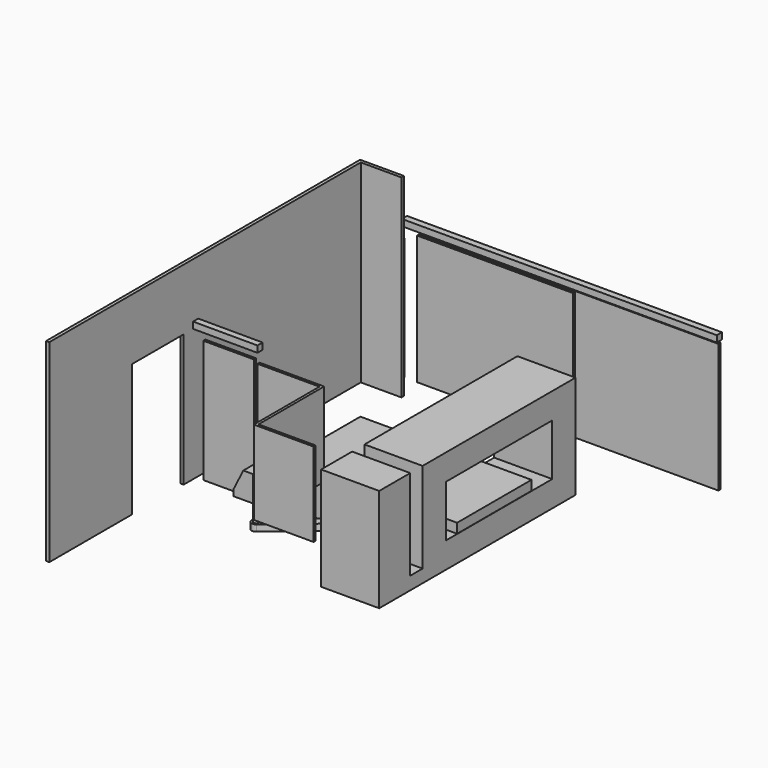
from build123d import *

# Parameters (mm, degrees)
F1_DEPTH  = 3000
F0_W      = 1150
F0_H      = 1440
F2_DEPTH  = 645
F0_W_2    = 900
F0_H_2    = 450
F0_W_3    = 660
F0_H_3    = 1290
F3_DEPTH  = 400
F4_DEPTH  = 1600
F5_W      = 900
F5_H      = 2960
F5_H_2    = 240
F5_H_3    = 600
F6_DEPTH  = 400
F7_W      = 1440
F7_H      = 150
F8_DEPTH  = 1500
F9_DEPTH  = 1400
F10_W     = 1000
F10_H     = 2050
F11_DEPTH = 50
F12_W     = 230
F12_H     = 200
F13_DEPTH = 350
F15_DEPTH = 100
F16_R     = 40
F17_DEPTH = 400
F18_W     = 300
F18_H     = 500
F19_DEPTH = 400
F20_SIZE2 = 300
F20_SIZE  = 150
F23_DEPTH = 1300
F24_W     = 2410
F24_H     = 40
F26_DEPTH = 2000
F29_DEPTH = 100
F28_W     = 4878.5563564301
F28_H     = 100
F24_W_2   = 40
F24_H_2   = 380
F30_DEPTH = 1900
F24_W_3   = 783


# Not quite as in the source:
# - the program builds the solid bodies; features that only make, move or delete a surface that nothing else refers to are left out


with BuildPart() as f1:
    # F0 (on Top) → F1 (new body)
    with BuildSketch(Plane.XY):
        Polygon((-2610, -3000), (-2560, -3000), (-2560, 3030), (-1930, 3030), (-1930, 3080), (-2610, 3080), (-2610, 3030), align=None)
    extrude(amount=F1_DEPTH)

    # F10 (on face) → F11 (cut, through all)
    with BuildSketch(Plane(origin=(-2610, 0, 0), x_dir=(0, -1, 0), z_dir=(-1, 0, 0))):
        with Locations((900, 1025)):
            Rectangle(F10_W, F10_H)
    extrude(amount=-F11_DEPTH, mode=Mode.SUBTRACT)

    # F28 (on offset) → F29 (join)
    with BuildSketch(Plane.XY.offset(2050)):
        Polygon((-1560, -220), (-1560, -120), (-2560, -117), (-2560, -217), align=None)
    extrude(amount=F29_DEPTH)

    # F24 (on Top) → F30 (join)
    with BuildSketch(Plane.XY):
        with Locations((-2248.5563564301, 3270)):
            Rectangle(F24_W_2, F24_H_2)
    extrude(amount=F30_DEPTH)


with BuildPart() as f2:
    # F0 (on Top) → F2 (new body)
    with BuildSketch(Plane.XY):
        with Locations((-655, 640)):
            Rectangle(F0_W, F0_H)
    extrude(amount=F2_DEPTH)

    # F7 (on face) → F8 (join)
    with BuildSketch(Plane.YZ.offset(-80)):
        with Locations((640, 570)):
            Rectangle(F7_W, F7_H)
    extrude(amount=F8_DEPTH)


with BuildPart() as f3:
    # F0 (on Top) → F3 (new body)
    with BuildSketch(Plane.XY):
        with Locations((860, 2125)):
            Rectangle(F0_W_2, F0_H_2)
        Polygon((1070, -80), (410, -80), (410, -160), (1310, -160), (1310, 1900), (410, 1900), (410, 1360), (1070, 1360), align=None)
        with Locations((740, 640)):
            Rectangle(F0_W_3, F0_H)
        with Locations((860, -805)):
            Rectangle(F0_W_2, F0_H_3)
    extrude(amount=F3_DEPTH)

    # F0 (on Top) → F4 (join)
    with BuildSketch(Plane.XY):
        with Locations((860, 2125)):
            Rectangle(F0_W_2, F0_H_2)
        with Locations((860, -805)):
            Rectangle(F0_W_2, F0_H_3)
    extrude(amount=F4_DEPTH)

    # F5 (on face) → F6 (join)
    with BuildSketch(Plane.XY.offset(1600)):
        with Locations((860, 870)):
            Rectangle(F5_W, F5_H)
        with Locations((860, -730)):
            Rectangle(F5_W, F5_H_2)
        with Locations((860, -1150)):
            Rectangle(F5_W, F5_H_3)
    extrude(amount=-F6_DEPTH)

    # F5 (on face) → F9 (cut)
    with BuildSketch(Plane.XY.offset(1600)):
        with Locations((860, -730)):
            Rectangle(F5_W, F5_H_2)
    extrude(amount=-F9_DEPTH, mode=Mode.SUBTRACT)

    # F12 (on face) → F13 (join)
    with BuildSketch(Plane(origin=(410, 0, 0), x_dir=(0, -1, 0), z_dir=(-1, 0, 0))):
        with Locations((445, 208.8655143976)):
            Rectangle(F12_W, F12_H)
    extrude(amount=F13_DEPTH)


with BuildPart() as f15:
    # F14 (on face) → F15 (new body)
    with BuildSketch(Plane.XY.offset(308.8655143976)):
        with BuildLine():
            Line((245.404305648, -449.7977561247), (161.8419163887, -350.2119785192))
            ThreePointArc((161.8419163887, -350.2119785192), (158.4474728868, -348.4449430772), (154.7977561247, -349.595694352))
            Line((154.7977561247, -349.595694352), (-821.908908852, -1169.1498967024))
            ThreePointArc((-821.908908852, -1169.1498967024), (-830.5368871923, -1267.7681403988), (-731.9186434959, -1276.396118739))
            Line((-731.9186434959, -1276.396118739), (244.7880214808, -456.8419163887))
            ThreePointArc((244.7880214808, -456.8419163887), (246.5550569228, -453.4474728868), (245.404305648, -449.7977561247))
        make_face()
    extrude(amount=F15_DEPTH)

    # F16 (on face) → F17 (join)
    with BuildSketch(Plane.XY.offset(408.8655143976)):
        with Locations((-776.913776174, -1222.7730077207)):
            Circle(F16_R)
    extrude(amount=F17_DEPTH)


with BuildPart() as f19:
    # F18 (on face) → F19 (new body)
    with BuildSketch(Plane.XY.offset(808.8655143976)):
        with Locations((-776.913776174, -1222.7730077207)):
            Rectangle(F18_W, F18_H)
    extrude(amount=F19_DEPTH)

    # F20
    f20_edges = [f19.edges().sort_by_distance(p)[0] for p in [
        (-926.913776, -1222.773008, 1208.865514),
    ]]
    f20_side = f19.faces().sort_by_distance((-776.913776, -1222.773008, 1208.865514))[0]
    chamfer(f20_edges, length=F20_SIZE, length2=F20_SIZE2, reference=f20_side)


with BuildPart() as f23:
    # F22 (on offset) → F23 (new body)
    with BuildSketch(Plane.XY.offset(600)):
        Polygon((324.4820666313, -1490), (324.4820666313, -1450), (-560, -1450), (-560, -180), (-1560, -180), (-1560, -220), (-600, -220), (-600, -1490), align=None)
    extrude(amount=F23_DEPTH)


with BuildPart() as f26:
    # F24 (on Top) → F26 (new body)
    with BuildSketch(Plane.XY):
        with Locations((-825, 3480)):
            Rectangle(F24_W, F24_H)
    extrude(amount=F26_DEPTH)


with BuildPart() as f26b:
    # F24 (on Top) → F26, piece 2 (new body)
    with BuildSketch(Plane.XY):
        with Locations((1385, 3540)):
            Rectangle(F24_W, F24_H)
    extrude(amount=F26_DEPTH)


with BuildPart() as f29:
    # F28 (on offset) → F29, piece 2 (new body)
    with BuildSketch(Plane.XY.offset(2050)):
        with Locations((170.721821785, 3510)):
            Rectangle(F28_W, F28_H)
    extrude(amount=F29_DEPTH)


with BuildPart() as f30:
    # F24 (on Top) → F30, piece 2 (new body)
    with BuildSketch(Plane.XY):
        with Locations((-2058.5, -137)):
            Rectangle(F24_W_3, F24_H)
    extrude(amount=F30_DEPTH)


solid = Compound([f1.part, f2.part, f3.part, f15.part, f19.part, f23.part, f26.part, f26b.part, f29.part, f30.part])
